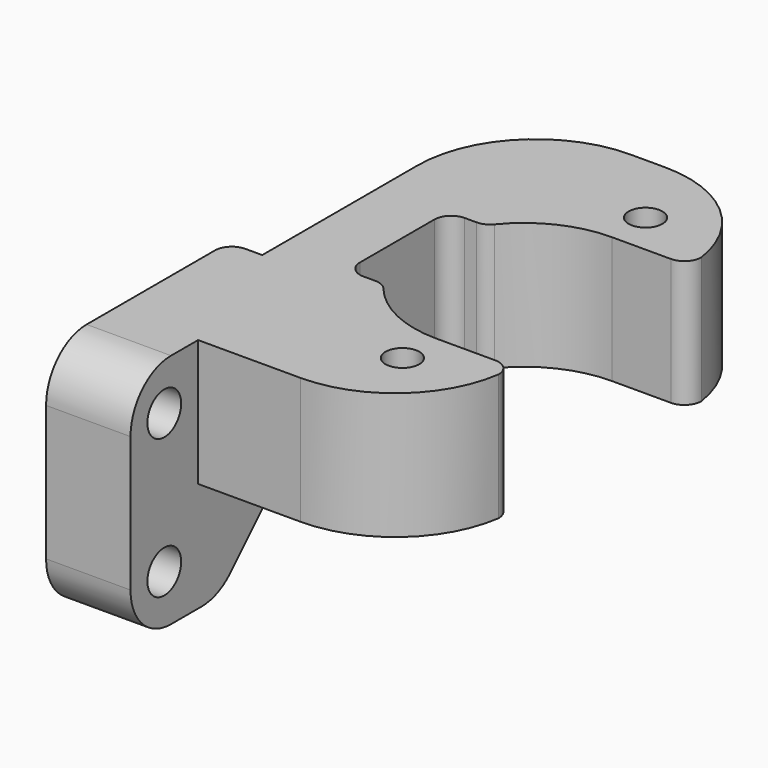
from build123d import *

# Parameters (mm, degrees)
F0_W          = 18
F0_H          = 32
F1_DEPTH      = 14
F2_W          = 13
F2_H          = 5
F2_W_2        = 2
F2_H_2        = 18.5
F3_DEPTH      = 14
F4_W          = 27
F4_H          = 6.5
F5_DEPTH      = 18.001
F6_R          = 1
F7_DEPTH      = 7.5
F8_R          = 1.25
F9_DEPTH      = 5
F10_T4_DEPTH  = 5
F11_T4_DEPTH  = 8.1066017178
F11_T9_DEPTH  = 8.1066017178
F11_T12_DEPTH = 20
F11_T14_DEPTH = 11.2132034356
F12_R         = 1
F13_T1_DEPTH  = 42.1410161514
F13_T3_DEPTH  = 42.5
F15_DEPTH     = 14.001
F16_R         = 1


# Not quite as in the source:
# - a fillet or chamfer that OpenCascade refuses, or shapes differently, is made with other operations: its cross-section is extruded or revolved along the edge and cut away or added


with BuildPart() as f1:
    # F0 (on Top) → F1 (new body)
    with BuildSketch(Plane.XY):
        with Locations((9, 16)):
            Rectangle(F0_W, F0_H)
    extrude(amount=F1_DEPTH)

    # F2 (on face) → F3 (cut, through all)
    with BuildSketch(Plane.XY.offset(14)):
        with Locations((11.5, 2.5)):
            Rectangle(F2_W, F2_H)
        with Locations((1, 22.75)):
            Rectangle(F2_W_2, F2_H_2)
    extrude(amount=-F3_DEPTH, mode=Mode.SUBTRACT)

    # F4 (on face) → F5 (cut, through all)
    with BuildSketch(Plane.YZ.offset(18)):
        with Locations((18.5, 3.25)):
            Rectangle(F4_W, F4_H)
    extrude(amount=-F5_DEPTH, mode=Mode.SUBTRACT)

    # F6 (on face) → F7 (cut, through all)
    with BuildSketch(Plane.XY.offset(14)):
        with Locations((13.5, 9.5)):
            Circle(F6_R)
        with BuildLine():
            ThreePointArc((18, 23.1904157598), (15.9251079936, 24.5306592691), (13.5, 25))
            ThreePointArc((13.5, 25), (7, 18.5), (13.5, 12))
            ThreePointArc((13.5, 12), (15.9251079936, 12.4693407309), (18, 13.8095842402))
            Line((18, 13.8095842402), (18, 23.1904157598))
        make_face()
        with Locations((13.5, 27.5)):
            Circle(F6_R)
        with BuildLine():
            Line((18, 25), (13.5, 25))
            ThreePointArc((13.5, 25), (15.9251079936, 24.5306592691), (18, 23.1904157598))
            Line((18, 23.1904157598), (18, 25))
        make_face()
        with BuildLine():
            ThreePointArc((18, 13.8095842402), (15.9251079936, 12.4693407309), (13.5, 12))
            Line((13.5, 12), (18, 12))
            Line((18, 12), (18, 13.8095842402))
        make_face()
    extrude(amount=-F7_DEPTH, mode=Mode.SUBTRACT)

    # F8 (on face) → F9 (cut, through all)
    with BuildSketch(Plane.YZ.offset(5)):
        with Locations((2.5, 11.2)):
            Circle(F8_R)
        with Locations((2.5, 2.95)):
            Circle(F8_R)
    extrude(amount=-F9_DEPTH, mode=Mode.SUBTRACT)

    # F10: chamfer of 8 on 1 edges, made by hand


with BuildPart() as f10_tool2:
    # F10_s3 → F10_t4 (new body)
    with BuildSketch(Plane.YZ.offset(5)):
        Polygon((5, -1.5), (13, 6.5), (5, 6.5), align=None)
    extrude(amount=-F10_T4_DEPTH)

    split(bisect_by=Plane.XY, keep=Keep.TOP)


with BuildPart() as f1_1:
    add(f1.part)

    # F10_t1: union F10_tool2
    add(f10_tool2.part)

    # F11: fillet of radius 3 on 5 edges, made by hand


with BuildPart() as f11_tool2:
    # F11_s3 → F11_t4 (new body)
    with BuildSketch(Plane.YZ.offset(5)):
        with BuildLine():
            ThreePointArc((14.2426406871, 6.5), (13.09459039, 6.2716385975), (12.1213203436, 5.6213203436))
            Line((12.1213203436, 5.6213203436), (13, 6.5))
            Line((13, 6.5), (14.2426406871, 6.5))
        make_face()
    extrude(amount=-F11_T4_DEPTH)

    split(bisect_by=Plane.YZ.offset(2), keep=Keep.TOP)


with BuildPart() as f1_2:
    add(f1_1.part)

    # F11_t1: union F11_tool2
    add(f11_tool2.part)


with BuildPart() as f11_tool7:
    # F11_s8 → F11_t9 (new body)
    with BuildSketch(Plane.YZ.offset(8.1066017178)):
        with BuildLine():
            ThreePointArc((14.2426406871, 6.5), (13.09459039, 6.2716385975), (12.1213203436, 5.6213203436))
            Line((12.1213203436, 5.6213203436), (13, 6.5))
            Line((13, 6.5), (14.2426406871, 6.5))
        make_face()
    extrude(amount=-F11_T9_DEPTH)

    split(bisect_by=Plane.YZ.offset(2), keep=Keep.BOTTOM)

    split(bisect_by=Plane.XZ.offset(-13.5), keep=Keep.TOP)


with BuildPart() as f1_3:
    add(f1_2.part)

    # F11_t6: union F11_tool7
    add(f11_tool7.part)

    # F11_s13 → F11_t12 (cut)
    with BuildSketch(Plane.YZ.offset(-7.5)):
        with BuildLine():
            ThreePointArc((0, 11), (0.8786796564, 13.1213203436), (3, 14))
            Line((3, 14), (0, 14))
            Line((0, 14), (0, 11))
        make_face()
        with BuildLine():
            ThreePointArc((0, 3), (0.8786796564, 0.8786796564), (3, 0))
            Line((3, 0), (0, 0))
            Line((0, 0), (0, 3))
        make_face()
    extrude(amount=F11_T12_DEPTH, mode=Mode.SUBTRACT)

    # F11_s15 → F11_t14 (cut)
    with BuildSketch(Plane.YZ.offset(-3.1066017178)):
        with BuildLine():
            ThreePointArc((7.3786796564, 0.8786796564), (6.40540961, 0.2283614025), (5.2573593129, 0))
            Line((5.2573593129, 0), (6.5, 0))
            Line((6.5, 0), (7.3786796564, 0.8786796564))
        make_face()
    extrude(amount=F11_T14_DEPTH, mode=Mode.SUBTRACT)

    # F12
    f12_edges = [f1_3.edges().sort_by_distance(p)[0] for p in [
        (18, 12, 10.25),
        (18, 25, 10.25),
    ]]
    fillet(f12_edges, radius=F12_R)

    # F13: fillet of radius 7 on 3 edges, made by hand

    # F13_s2 → F13_t1 (cut)
    with BuildSketch(Plane.XY.offset(-10.8205080757)):
        with BuildLine():
            ThreePointArc((18, 11), (15.6543724647, 6.7084973779), (11.0717967697, 5))
            Line((11.0717967697, 5), (11.0717967697, 4.86))
            Line((11.0717967697, 4.86), (18, 4.86))
            Line((18, 4.86), (18.14, 5))
            ThreePointArc((18.14, 5), (18.14, 8), (18.1385640646, 10.98))
            Line((18.1385640646, 10.98), (18, 11))
        make_face()
        with BuildLine():
            ThreePointArc((18, 26), (15.6543724647, 30.2915026221), (11.0717967697, 32))
            Line((11.0717967697, 32), (11.0717967697, 32.14))
            Line((11.0717967697, 32.14), (18, 32.14))
            Line((18, 32.14), (18.14, 32))
            ThreePointArc((18.14, 32), (18.14, 29), (18.1385640646, 26.02))
            Line((18.1385640646, 26.02), (18, 26))
        make_face()
    extrude(amount=F13_T1_DEPTH, mode=Mode.SUBTRACT)

    # F13_s4 → F13_t3 (cut)
    with BuildSketch(Plane.XY.offset(-11)):
        with BuildLine():
            ThreePointArc((9, 32), (4.0502525317, 29.9497474683), (2, 25))
            Line((2, 25), (1.86, 25))
            Line((1.86, 25), (1.86, 32.14))
            Line((1.86, 32.14), (9, 32.14))
            Line((9, 32.14), (9, 32))
        make_face()
    extrude(amount=F13_T3_DEPTH, mode=Mode.SUBTRACT)

    # F14 (on face) → F15 (cut, through all)
    with BuildSketch(Plane.XY.offset(14)):
        with BuildLine():
            ThreePointArc((8.1908098546, 14.75), (7, 18.5), (8.1908098546, 22.25))
            Line((8.1908098546, 22.25), (5.9908098546, 22.25))
            Line((5.9908098546, 22.25), (5.9908098546, 14.75))
            Line((5.9908098546, 14.75), (8.1908098546, 14.75))
        make_face()
    extrude(amount=-F15_DEPTH, mode=Mode.SUBTRACT)

    # F16
    f16_edges = [f1_3.edges().sort_by_distance(p)[0] for p in [
        (5.99081, 14.75, 10.25),
        (5.99081, 22.25, 10.25),
        (8.19081, 22.25, 10.25),
        (8.19081, 14.75, 10.25),
        (0, 13.5, 10.203314),
    ]]
    fillet(f16_edges, radius=F16_R)


solid = f1_3.part
